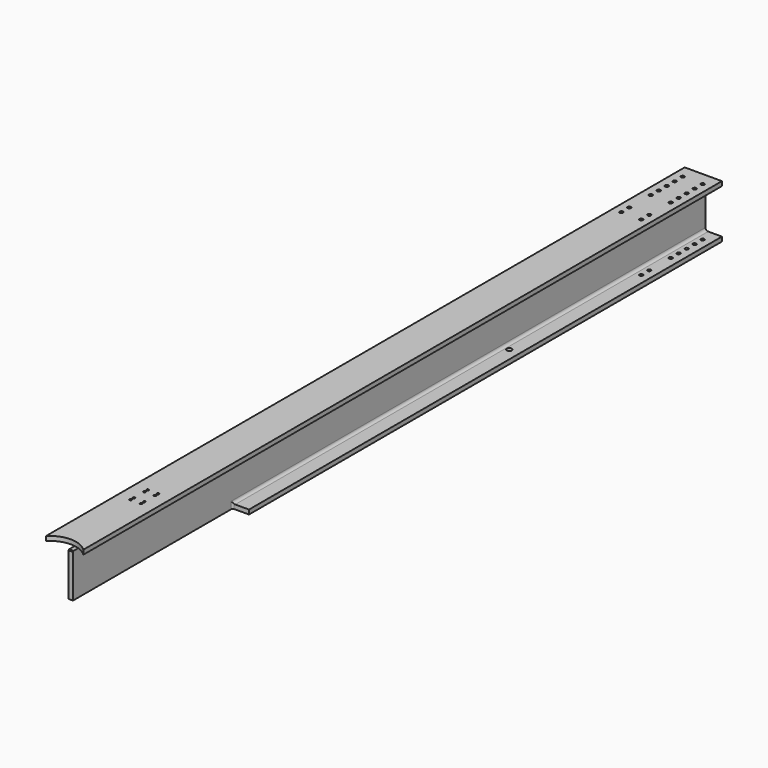
from build123d import *

# Parameters (mm, degrees)
F1_DEPTH  = 1524
F2_R      = 5.08
F4_DEPTH  = 101.6
F6_W      = 48.26
F6_H      = 10.16
F7_DEPTH  = 12.7
F8_SIZE   = 1.27
F10_D     = 4.318
F10_DEPTH = 25.4
F10_TIP   = 1.2972580765
F11_W     = 35.4891605821
F11_H     = 399.7617846188
F12_DEPTH = 25.4
F13_R     = 3.175
F15_D     = 9.8044
F15_DEPTH = 25.4
F15_TIP   = 2.9455389266
F17_D     = 6.5278
F19_D     = 6.35


# Not quite as in the source:
# - a pattern or mirror of a feature is missing from the dataset's text; its kind, count and spacing are read off the source's solid


with BuildPart() as f1:
    # F0 (on Front) → F1 (new body)
    with BuildSketch(Plane.XZ):
        Polygon((-35.56, -50.8), (35.56, -50.8), (35.56, -42.418), (4.191, -42.418), (4.191, 0), (4.191, 42.418), (35.56, 42.418), (35.56, 50.8), (0, 50.8), (-4.191, 50.8), (-35.56, 50.8), (-35.56, 42.418), (-4.191, 42.418), (-4.191, 0), (-4.191, -42.418), (-35.56, -42.418), align=None)
    extrude(amount=F1_DEPTH)

    # F2
    f2_edges = [f1.edges().sort_by_distance(p)[0] for p in [
        (4.191, -762, 42.418),
        (4.191, -762, -42.418),
        (-4.191, -762, -42.418),
        (-4.191, -762, 42.418),
    ]]
    fillet(f2_edges, radius=F2_R)

    # F3 (on face) → F4 (cut)
    with BuildSketch(Plane.XY.offset(50.8)):
        Polygon((35.56, -1524), (0, -1524), (0, -1560.278456417), align=None)
        with BuildLine():
            Line((0, -1560.278456417), (0, -1524))
            Line((0, -1524), (-35.56, -1524))
            ThreePointArc((-35.56, -1524), (-47.0297011791, -1579.4838516748), (0, -1611.078456417))
            ThreePointArc((0, -1611.078456417), (35.9210244843, -1596.1994809013), (50.8, -1560.278456417))
            ThreePointArc((50.8, -1560.278456417), (46.835285843, -1540.6037010183), (35.56, -1524))
            Line((35.56, -1524), (0, -1560.278456417))
        make_face()
        with BuildLine():
            Line((-35.56, -1524), (0, -1524))
            Line((0, -1524), (35.56, -1524))
            ThreePointArc((35.56, -1524), (0, -1509.478456417), (-35.56, -1524))
        make_face()
    extrude(amount=-F4_DEPTH, mode=Mode.SUBTRACT)

    # F6 (on face) → F7 (cut, symmetric)
    with BuildSketch(Plane.YZ.offset(4.191)):
        with Locations((-1486.2015990684, 37.338)):
            Rectangle(F6_W, F6_H)
    extrude(amount=F7_DEPTH, both=True, mode=Mode.SUBTRACT)

    # F8
    f8_edges = [f1.edges().sort_by_distance(p)[0] for p in [
        (0, -1509.478456, 32.258),
    ]]
    chamfer(f8_edges, length=F8_SIZE)

    # F10
    with Locations(Plane.XY.offset(50.8)):
        with Locations((-10.2286281229, -1353.8202740377), (-10.2286199642, -1346.2002740377), (-10.2286199642, -1320.8002740377), (-10.2286381092, -1313.1802740377), (9.711437429, -1313.1802740377), (9.711419284, -1320.8002740377), (9.711419284, -1346.2002740377), (9.7114274426, -1353.8202740377)):
            Hole(F10_D / 2, depth=F10_DEPTH)
            with Locations((0, 0, -(F10_DEPTH + F10_TIP / 2))):  # 118° drill point
                Cone(0, F10_D / 2, F10_TIP, mode=Mode.SUBTRACT)

    # F11 (on face) → F12 (cut)
    with BuildSketch(Plane(origin=(0, 0, -50.8), x_dir=(1, 0, 0), z_dir=(0, 0, -1))):
        Polygon((4.191, 1528.4134149551), (4.191, 1509.6516303364), (4.191, 1128.6516303364), (39.6801605821, 1128.6516303364), (39.6801605821, 1528.4134149551), align=None)
        with Locations((-21.935580291, 1328.5325226457)):
            Rectangle(F11_W, F11_H)
    extrude(amount=-F12_DEPTH, mode=Mode.SUBTRACT)

    # F13
    f13_edges = [f1.edges().sort_by_distance(p)[0] for p in [
        (4.191, -1128.65163, -44.069),
        (-4.191, -1128.65163, -44.069),
    ]]
    fillet(f13_edges, radius=F13_R)

    # F15
    with Locations(Plane(origin=(0, 0, -50.8), x_dir=(1, 0, 0), z_dir=(0, 0, -1))):
        with Locations((15.875, 482.6), (-15.875, 482.6)):
            Hole(F15_D / 2, depth=F15_DEPTH)
            with Locations((0, 0, -(F15_DEPTH + F15_TIP / 2))):  # 118° drill point
                Cone(0, F15_D / 2, F15_TIP, mode=Mode.SUBTRACT)

    # F17 (through all)
    with Locations(Plane.XY.offset(50.8)):
        with Locations((-19.05, -82.55), (-19.05, -101.6), (-19.05, -63.5), (-19.05, -44.45), (-19.05, -25.4), (19.05, -25.4), (19.05, -44.45), (19.05, -63.5), (19.05, -101.6), (19.05, -101.6)):
            f17 = Hole(F17_D / 2)

    # F17_copies: F17 across plane
    add(f17.mirror(Plane(origin=(0, 0, 0), x_dir=(0, 0, 1), z_dir=(1, 0, 0))), mode=Mode.SUBTRACT)

    # F19 (through all)
    with Locations(Plane.XY.offset(50.8)):
        with Locations((-19.05, -152.8064), (-19.05, -171.8564), (19.05, -152.8064), (19.05, -171.8564)):
            Hole(F19_D / 2)


solid = f1.part
